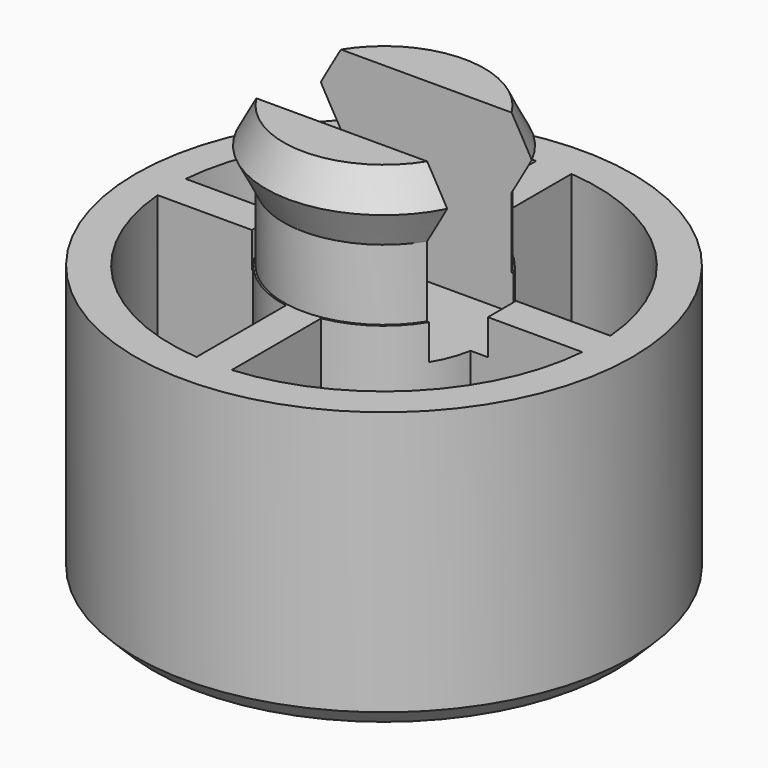
from build123d import *

# Parameters (mm, degrees)
F0_R       = 14.1
F1_DEPTH   = 16
F2_SIZE    = 1
F3_R       = 5.7
F4_DEPTH   = 8
F5_R       = 6.7
F5_R_2     = 5.7
F6_DEPTH   = 4
F7_SIZE2   = 2
F7_SIZE    = 1
F7_2_SIZE2 = 1.99999
F7_2_SIZE  = 0.99999
F8_W       = 13.4
F8_H       = 6
F9_DEPTH   = 10


# Not quite as in the source:
# - a fillet or chamfer is up to 0.001 mm smaller than in the source, because OpenCascade refuses the exact size


with BuildPart() as f1:
    # F0 (on Top) → F1 (new body)
    with BuildSketch(Plane.XY):
        Circle(F0_R)
        with BuildLine():
            Line((-12.0586068847, -1), (-5.7131427428, -1))
            ThreePointArc((-5.7131427428, -1), (-4.1012193309, -4.1012193309), (-1, -5.7131427428))
            Line((-1, -5.7131427428), (-1, -12.0586068847))
            ThreePointArc((-1, -12.0586068847), (-8.5559920524, -8.5559920524), (-12.0586068847, -1))
        make_face(mode=Mode.SUBTRACT)
        with BuildLine():
            ThreePointArc((12.0586068847, -1), (8.5559920524, -8.5559920524), (1, -12.0586068847))
            Line((1, -12.0586068847), (1, -5.7131427428))
            ThreePointArc((1, -5.7131427428), (4.1012193309, -4.1012193309), (5.7131427428, -1))
            Line((5.7131427428, -1), (12.0586068847, -1))
        make_face(mode=Mode.SUBTRACT)
        with BuildLine():
            ThreePointArc((-12.0586068847, 1), (-8.5559920524, 8.5559920524), (-1, 12.0586068847))
            Line((-1, 12.0586068847), (-1, 5.7131427428))
            ThreePointArc((-1, 5.7131427428), (-4.1012193309, 4.1012193309), (-5.7131427428, 1))
            Line((-5.7131427428, 1), (-12.0586068847, 1))
        make_face(mode=Mode.SUBTRACT)
        with BuildLine():
            Line((12.0586068847, 1), (5.7131427428, 1))
            ThreePointArc((5.7131427428, 1), (4.1012193309, 4.1012193309), (1, 5.7131427428))
            Line((1, 5.7131427428), (1, 12.0586068847))
            ThreePointArc((1, 12.0586068847), (8.5559920524, 8.5559920524), (12.0586068847, 1))
        make_face(mode=Mode.SUBTRACT)
    extrude(amount=F1_DEPTH)

    # F2
    f2_edges = [f1.edges().sort_by_distance(p)[0] for p in [
        (-14.1, 0, 0),
    ]]
    chamfer(f2_edges, length=F2_SIZE)

    # F3 (on face) → F4 (join)
    with BuildSketch(Plane.XY.offset(16)):
        Circle(F3_R)
    extrude(amount=F4_DEPTH)

    # F5 (on face) → F6 (join)
    with BuildSketch(Plane.XY.offset(24)):
        Circle(F5_R)
        Circle(F5_R_2, mode=Mode.SUBTRACT)
    extrude(amount=-F6_DEPTH)

    # F7
    f7_edges = [f1.edges().sort_by_distance(p)[0] for p in [
        (-6.7, 0, 24),
    ]]
    f7_side = f1.faces().sort_by_distance((0, 0, 24))[0]
    chamfer(f7_edges, length=F7_SIZE, length2=F7_SIZE2, reference=f7_side)

    # F7#2 (size 1 and 2 in the source; OpenCascade refuses exactly that, so slightly less here)
    f7_2_edges = [f1.edges().sort_by_distance(p)[0] for p in [
        (-6.7, 0, 20),
    ]]
    f7_2_side = f1.faces().sort_by_distance((-6.510495, 0, 20))[0]
    chamfer(f7_2_edges, length=F7_2_SIZE, length2=F7_2_SIZE2, reference=f7_2_side)

    # F8 (on face) → F9 (cut)
    with BuildSketch(Plane.XY.offset(24)):
        Rectangle(F8_W, F8_H)
    extrude(amount=-F9_DEPTH, mode=Mode.SUBTRACT)


solid = f1.part
